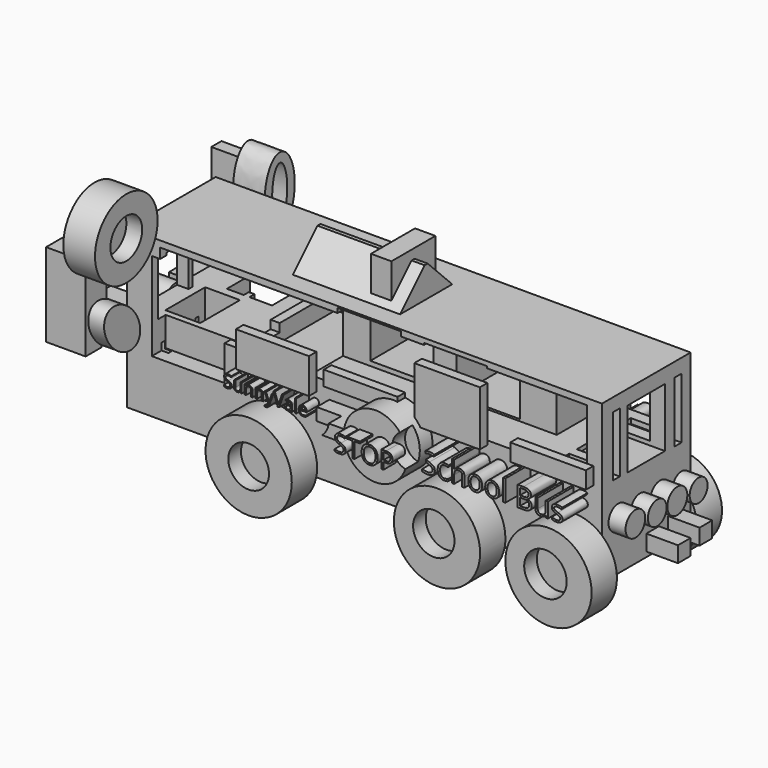
from build123d import *

# Parameters (mm, degrees)
F0_W          = 381
F0_H          = 126.5198698357
F1_DEPTH      = 88.9
F2_W          = 50.8
F2_H          = 50.8
F3_DEPTH      = 127
F4_W          = 50.8
F4_H          = 50.8
F5_DEPTH      = 125.476
F6_W          = 50.8
F6_H          = 50.8
F7_DEPTH      = 353.06
F8_W          = 50.8
F8_H          = 50.8
F9_DEPTH      = 348.996
F10_W         = 36.2219065428
F10_H         = 82.3675262787
F11_DEPTH     = 23.368
F12_W         = 77.2041911259
F12_H         = 49.2639932781
F13_DEPTH     = 88.9
F14_R         = 31.7675639144
F15_DEPTH     = 25.4
F16_R         = 34.5900274771
F17_DEPTH     = 25.4
F18_R         = 34.5948
F19_DEPTH     = 25.4
F20_R         = 34.5948
F21_DEPTH     = 25.4
F22_R         = 34.5948
F23_DEPTH     = 25.4
F24_R         = 34.5948
F25_DEPTH     = 25.4
F26_W         = 58.3547353745
F26_H         = 70.7532842644
F27_DEPTH     = 13.97
F28_W         = 86.0774414614
F28_H         = 53.8219604641
F29_DEPTH     = 24.638
F30_W         = 16.3701735437
F30_H         = 44.1550221294
F31_DEPTH     = 7.62
F32_W         = 12.7
F32_H         = 12.7
F33_DEPTH     = 25.4
F34_W         = 12.7
F34_H         = 12.7
F35_DEPTH     = 25.4
F36_W         = 61.9277469814
F36_H         = 34.5999319106
F37_DEPTH     = 25.4
F38_W         = 4.6026781201
F38_H         = 70.9157045931
F39_DEPTH     = 5.08
F40_W         = 4.1819550097
F40_H         = 60.264851898
F41_DEPTH     = 9.144
F42_W         = 32.3324687779
F42_H         = 9.9669089541
F43_DEPTH     = 25.4
F44_R         = 25.4464837563
F45_DEPTH     = 25.4
F46_W         = 50.8
F46_H         = 5.08
F47_DEPTH     = 25.4
F48_W         = 10.16
F48_H         = 76.2
F49_DEPTH     = 25.4
F51_DEPTH     = 25.4
F52_W         = 142.2856748104
F52_H         = 27.6914052665
F53_DEPTH     = 19.05
F54_R         = 18.3963073453
F55_T4_DEPTH  = 267.5098197727
F56_R         = 9.8577445276
F56_R_2       = 9.3926475971
F56_R_3       = 10.0311781721
F56_R_4       = 8.995280697
F57_DEPTH     = 13.716
F58_T4_DEPTH  = 216.7189372501
F58_T11_DEPTH = 216.7189372501
F58_T17_DEPTH = 216.7189372501
F58_T25_DEPTH = 216.7189372501
F58_T32_DEPTH = 216.7189372501
F59_T4_DEPTH  = 216.7189372501
F59_T10_DEPTH = 216.7189372501
F59_T17_DEPTH = 216.7189372501
F59_T25_DEPTH = 216.7189372501
F59_T31_DEPTH = 216.7189372501
F60_W         = 7.0483535528
F60_H         = 48.1858924031
F60_W_2       = 37.5115424395
F60_H_2       = 47.3481267691
F60_W_3       = 7.0474697277
F60_H_3       = 48.6524347216
F61_DEPTH     = 40.64
F62_W         = 2.7957055718
F62_H         = 33.0349653959
F62_W_2       = 2.7912929654
F62_H_2       = 33.7924696505
F62_W_3       = 2.7886535972
F62_H_3       = 35.0428596139
F62_W_4       = 3.2654814422
F62_H_4       = 35.3162623942
F62_W_5       = 3.2645985484
F62_H_5       = 37.0068624616
F62_W_6       = 3.2628290355
F62_H_6       = 37.7731472254
F62_W_7       = 3.7387758493
F62_H_7       = 37.1046811342
F62_W_8       = 3.2584369183
F62_H_8       = 39.2618253827
F63_DEPTH     = 25.4
F64_R         = 10.9485201538
F65_DEPTH     = 25.4
F66_TEXT_SIZE = 19.9620301525
F67_DEPTH     = 25.4
F68_TEXT_SIZE = 13.9440008853
F69_DEPTH     = 12.7
F70_TEXT_SIZE = 22.4992270685
F71_DEPTH     = 25.4
F72_TEXT_SIZE = 19.452727348
F73_DEPTH     = 12.7
F74_W         = 64.9670958519
F74_H         = 13.338890858
F75_DEPTH     = 31.75
F76_W         = 31.75
F76_H         = 20.7315831661
F77_DEPTH     = 53.594
F78_R         = 31.3869658327
F79_DEPTH     = 25.4
F80_R         = 16.3249163215
F80_R_2       = 16.6206391451
F80_R_3       = 17.0464544412
F80_R_4       = 14.0490359697
F80_R_5       = 15.6096867974
F80_R_6       = 13.548085848
F81_DEPTH     = 12.7
F82_R         = 15.1490274208
F82_R_2       = 15.5967239553
F82_R_3       = 14.1064228958
F83_DEPTH     = 12.7
F84_W         = 68.6886934564
F84_H         = 34.0798477687
F85_DEPTH     = 20.32
F86_R         = 8.4618533599
F87_DEPTH     = 12.7
F88_W         = 58.5370287299
F88_H         = 28.1933201477
F88_W_2       = 59.2209338211
F88_H_2       = 11.8853002787
F88_W_3       = 52.6049807668
F88_H_3       = 43.9174287021
F88_W_4       = 60.577660799
F88_H_4       = 13.7192141265
F89_DEPTH     = 7.62
F90_R         = 12.6748476443
F91_DEPTH     = 7.62
F92_W         = 32.9182857215
F92_H         = 50.8
F93_DEPTH     = 291.846
F94_W         = 55.9817142785
F94_H         = 15.9087059989
F95_DEPTH     = 230.378
F96_W         = 27.9357880354
F96_H         = 39.8813150823
F97_DEPTH     = 25.4
F98_W         = 4.846972879
F98_H         = 34.0798477687
F99_DEPTH     = 25.4
F100_R        = 5.4790358638
F101_DEPTH    = 25.4
F102_R        = 15.9473548046
F103_DEPTH    = 12.7
F105_DEPTH    = 12.7
F106_W        = 7.8915469348
F106_H        = 8.9074093848
F106_W_2      = 8.1563740969
F106_H_2      = 9.9165849388
F107_DEPTH    = 12.7
F109_DEPTH    = 12.7


# Not quite as in the source:
# - a fillet or chamfer that OpenCascade refuses, or shapes differently, is made with other operations: its cross-section is extruded or revolved along the edge and cut away or added
# - Text() gives the source's letters only with a copy of the font that has no kerning and outlines rounded to 1/6400 em; it was checked with that copy


with BuildPart() as f1:
    # F0 (on Front) → F1 (new body)
    with BuildSketch(Plane.XZ):
        with Locations((-29.1106849909, 15.0728300214)):
            Rectangle(F0_W, F0_H)
    extrude(amount=F1_DEPTH)

    # F2 (on face) → F3 (cut)
    with BuildSketch(Plane(origin=(0, 0, 0), x_dir=(-1, 0, 0), z_dir=(0, 1, 0))):
        with Locations((-124.1777315736, 47.8980025902)):
            Rectangle(F2_W, F2_H)
    extrude(amount=-F3_DEPTH, mode=Mode.SUBTRACT)

    # F4 (on face) → F5 (cut)
    with BuildSketch(Plane.XZ.offset(88.9)):
        with Locations((43.9449427649, 49.4133692031)):
            Rectangle(F4_W, F4_H)
    extrude(amount=-F5_DEPTH, mode=Mode.SUBTRACT)

    # F6 (on face) → F7 (cut)
    with BuildSketch(Plane(origin=(0, 0, 0), x_dir=(-1, 0, 0), z_dir=(0, 1, 0))):
        with Locations((25.4, 51.5604968276)):
            Rectangle(F6_W, F6_H)
    extrude(amount=-F7_DEPTH, mode=Mode.SUBTRACT)

    # F8 (on face) → F9 (cut)
    with BuildSketch(Plane(origin=(0, 0, 0), x_dir=(-1, 0, 0), z_dir=(0, 1, 0))):
        with Locations((98.0433411896, 40.8556130676)):
            Rectangle(F8_W, F8_H)
    extrude(amount=-F9_DEPTH, mode=Mode.SUBTRACT)

    # F10 (on face) → F11 (cut)
    with BuildSketch(Plane(origin=(0, 0, 0), x_dir=(-1, 0, 0), z_dir=(0, 1, 0))):
        with Locations((173.8056764007, -7.0033417571)):
            Rectangle(F10_W, F10_H)
    extrude(amount=-F11_DEPTH, mode=Mode.SUBTRACT)

    # F12 (on face) → F13 (cut)
    with BuildSketch(Plane(origin=(-219.6106849909, 0, 0), x_dir=(0, -1, 0), z_dir=(-1, 0, 0))):
        with Locations((43.8935565762, 42.518469505)):
            Rectangle(F12_W, F12_H)
    extrude(amount=-F13_DEPTH, mode=Mode.SUBTRACT)

    # F14 (on face) → F15 (join)
    with BuildSketch(Plane(origin=(0, 0, 0), x_dir=(-1, 0, 0), z_dir=(0, 1, 0))):
        with Locations((-134.4692409039, -42.1050563455)):
            Circle(F14_R)
    extrude(amount=F15_DEPTH)

    # F16 (on face) → F17 (join)
    with BuildSketch(Plane(origin=(0, 0, 0), x_dir=(-1, 0, 0), z_dir=(0, 1, 0))):
        with Locations((-54.2609095573, -41.1995537579)):
            Circle(F16_R)
    extrude(amount=F17_DEPTH)

    # F18 (on face) → F19 (join)
    with BuildSketch(Plane(origin=(0, 0, 0), x_dir=(-1, 0, 0), z_dir=(0, 1, 0))):
        with Locations((101.8479317427, -41.1263331771)):
            Circle(F18_R)
    extrude(amount=F19_DEPTH)

    # F20 (on face) → F21 (join)
    with BuildSketch(Plane.XZ.offset(88.9)):
        with Locations((138.8085335493, -40.9661456943)):
            Circle(F20_R)
    extrude(amount=F21_DEPTH)

    # F22 (on face) → F23 (join)
    with BuildSketch(Plane.XZ.offset(88.9)):
        with Locations((49.349758774, -42.1094596386)):
            Circle(F22_R)
    extrude(amount=F23_DEPTH)

    # F24 (on face) → F25 (join)
    with BuildSketch(Plane.XZ.offset(88.9)):
        with Locations((-101.7133966088, -41.3157492876)):
            Circle(F24_R)
    extrude(amount=F25_DEPTH)

    # F26 (on face) → F27 (cut)
    with BuildSketch(Plane.XZ.offset(88.9)):
        with Locations((-170.5612689257, 29.7877525445)):
            Rectangle(F26_W, F26_H)
    extrude(amount=-F27_DEPTH, mode=Mode.SUBTRACT)

    # F28 (on face) → F29 (join)
    with BuildSketch(Plane.XY.offset(78.3327649392)):
        with Locations((-56.0307926498, -47.2026942298)):
            Rectangle(F28_W, F28_H)
    extrude(amount=F29_DEPTH)

    # F30 (on face) → F31 (join)
    with BuildSketch(Plane.XY.offset(102.9707649392)):
        with Locations((-31.680950895, -46.8696849421)):
            Rectangle(F30_W, F30_H)
    extrude(amount=F31_DEPTH)

    # F32 (on face) → F33 (join)
    with BuildSketch(Plane.YZ.offset(161.3893150091)):
        with Locations((-16.4386960678, -34.2422378585)):
            Rectangle(F32_W, F32_H)
    extrude(amount=F33_DEPTH)

    # F34 (on face) → F35 (join)
    with BuildSketch(Plane.YZ.offset(161.3893150091)):
        with Locations((-38.1, -37.8550173879)):
            Rectangle(F34_W, F34_H)
    extrude(amount=F35_DEPTH)

    # F36 (on face) → F37 (cut)
    with BuildSketch(Plane(origin=(-130.7106849909, 0, 0), x_dir=(0, -1, 0), z_dir=(-1, 0, 0))):
        with Locations((40.43697007, 46.5236147866)):
            Rectangle(F36_W, F36_H)
    extrude(amount=-F37_DEPTH, mode=Mode.SUBTRACT)

    # F38 (on face) → F39 (join)
    with BuildSketch(Plane(origin=(0, -23.368, 0), x_dir=(-1, 0, 0), z_dir=(0, 1, 0))):
        with Locations((176.1070154607, -17.5713794306)):
            Rectangle(F38_W, F38_H)
    extrude(amount=F39_DEPTH)

    # F40 (on face) → F41 (join)
    with BuildSketch(Plane(origin=(-219.6106849909, 0, 0), x_dir=(0, -1, 0), z_dir=(-1, 0, 0))):
        with Locations((36.5860965103, 42.0981813222)):
            Rectangle(F40_W, F40_H)
    extrude(amount=-F41_DEPTH)

    # F42 (on face) → F43 (join)
    with BuildSketch(Plane.XZ.offset(88.9)):
        with Locations((-41.1809217185, 4.983454477)):
            Rectangle(F42_W, F42_H)
    extrude(amount=F43_DEPTH)

    # F44 (on face) → F45 (join)
    with BuildSketch(Plane.XZ.offset(88.9)):
        with Locations((0, 6.0606561601)):
            Circle(F44_R)
    extrude(amount=F45_DEPTH)

    # F46 (on face) → F47 (join)
    with BuildSketch(Plane(origin=(-219.6106849909, 0, 0), x_dir=(0, -1, 0), z_dir=(-1, 0, 0))):
        with Locations((-10.1813804358, 6.5084572987)):
            Rectangle(F46_W, F46_H)
    extrude(amount=F47_DEPTH)

    # F48 (on face) → F49 (join)
    with BuildSketch(Plane(origin=(-245.0106849909, 0, 0), x_dir=(0, -1, 0), z_dir=(-1, 0, 0))):
        with Locations((-32.4664697665, 42.0684572987)):
            Rectangle(F48_W, F48_H)
    extrude(amount=-F49_DEPTH)

    # F50 (on face) → F51 (join)
    with BuildSketch(Plane.YZ.offset(-219.6106849909)):
        with BuildLine():
            add(Edge.make_bspline(
                [(32.4664697665, 90.7859504223), (6.4393695077, 90.7859504223), (19.4529196371, 49.0357801318), (32.4664697665, 7.2856098413), (45.4800198959, 49.0357801318), (58.4935700253, 90.7859504223), (32.4664697665, 90.7859504223)],
                knots=[0, 0, 0, 2.0943951024, 2.0943951024, 4.1887902048, 4.1887902048, 6.2831853072, 6.2831853072, 6.2831853072], degree=2, weights=[1, 0.5, 1, 0.5, 1, 0.5, 1]))
        make_face()
    extrude(amount=F51_DEPTH)

    # F52 (on face) → F53 (join)
    with BuildSketch(Plane(origin=(0, 0, -48.1871048965), x_dir=(1, 0, 0), z_dir=(0, 0, -1))):
        with Locations((71.1428374052, 47.2517032176)):
            Rectangle(F52_W, F52_H)
    extrude(amount=F53_DEPTH)

    # F54
    f54_edges = [f1.edges().sort_by_distance(p)[0] for p in [
        (142.285675, -47.251703, -67.237105),
    ]]
    fillet(f54_edges, radius=F54_R)

    # F55: fillet of radius 69.9059679121 on 1 edges, made by hand


with BuildPart() as f55_tool2:
    # F55_s3 → F55_t4 (new body)
    with BuildSketch(Plane.XZ.offset(181.006613104)):
        with BuildLine():
            ThreePointArc((47.9636829012, -67.2371048965), (22.1595292751, -62.3002835492), (0, -48.1871048965))
            Line((0, -48.1871048965), (0, -67.2371048965))
            Line((0, -67.2371048965), (47.9636829012, -67.2371048965))
        make_face()
    extrude(amount=-F55_T4_DEPTH)

    split(bisect_by=Plane.XZ.offset(88.9), keep=Keep.BOTTOM)

    split(bisect_by=Plane.XZ, keep=Keep.TOP)


with BuildPart() as f1_1:
    add(f1.part)

    # F55_t1: cut F55_tool2
    add(f55_tool2.part, mode=Mode.SUBTRACT)

    # F56 (on face) → F57 (join)
    with BuildSketch(Plane.YZ.offset(161.3893150091)):
        with Locations((-72.517581284, -8.7204622105)):
            Circle(F56_R)
        with Locations((-50.6030321121, -9.8998090252)):
            Circle(F56_R_2)
        with Locations((-30.4931569844, -9.6532292664)):
            Circle(F56_R_3)
        with Locations((-9.1150775552, -10.8976587653)):
            Circle(F56_R_4)
    extrude(amount=F57_DEPTH)

    # F58: chamfer of 25.4 on 1 edges, made by hand


with BuildPart() as f58_tool2:
    # F58_s3 → F58_t4 (new body)
    with BuildSketch(Plane.YZ.offset(-164.3902612749)):
        Polygon((-74.1136744618, 77.5707649392), (-48.7136744618, 102.9707649392), (-74.1136744618, 102.9707649392), align=None)
    extrude(amount=F58_T4_DEPTH)

    split(bisect_by=Plane.XY.offset(78.3327649392), keep=Keep.TOP)

    split(bisect_by=Plane.YZ.offset(-39.8660376668), keep=Keep.BOTTOM)

    split(bisect_by=Plane.XZ.offset(68.9471960068), keep=Keep.TOP)


with BuildPart() as f1_2:
    add(f1_1.part)

    # F58_t1: cut F58_tool2
    add(f58_tool2.part, mode=Mode.SUBTRACT)


with BuildPart() as f58_tool9:
    # F58_s10 → F58_t11 (new body)
    with BuildSketch(Plane.YZ.offset(-164.3902612749)):
        Polygon((-74.1136744618, 77.5707649392), (-48.7136744618, 102.9707649392), (-74.1136744618, 102.9707649392), align=None)
    extrude(amount=F58_T11_DEPTH)

    split(bisect_by=Plane.YZ.offset(-39.8660376668), keep=Keep.BOTTOM)

    split(bisect_by=Plane.XZ.offset(68.9471960068), keep=Keep.BOTTOM)


with BuildPart() as f1_3:
    add(f1_2.part)

    # F58_t8: cut F58_tool9
    add(f58_tool9.part, mode=Mode.SUBTRACT)


with BuildPart() as f58_tool15:
    # F58_s16 → F58_t17 (new body)
    with BuildSketch(Plane.YZ.offset(-164.3902612749)):
        Polygon((-74.1136744618, 77.5707649392), (-48.7136744618, 102.9707649392), (-74.1136744618, 102.9707649392), align=None)
    extrude(amount=F58_T17_DEPTH)

    split(bisect_by=Plane.XY.offset(78.3327649392), keep=Keep.TOP)

    split(bisect_by=Plane.YZ.offset(-39.8660376668), keep=Keep.TOP)

    split(bisect_by=Plane.XZ.offset(68.9471960068), keep=Keep.TOP)

    split(bisect_by=Plane.YZ.offset(-23.4958641231), keep=Keep.BOTTOM)


with BuildPart() as f1_4:
    add(f1_3.part)

    # F58_t14: cut F58_tool15
    add(f58_tool15.part, mode=Mode.SUBTRACT)


with BuildPart() as f58_tool23:
    # F58_s24 → F58_t25 (new body)
    with BuildSketch(Plane.YZ.offset(-164.3902612749)):
        Polygon((-74.1136744618, 77.5707649392), (-48.7136744618, 102.9707649392), (-74.1136744618, 102.9707649392), align=None)
    extrude(amount=F58_T25_DEPTH)

    split(bisect_by=Plane.XY.offset(78.3327649392), keep=Keep.TOP)

    split(bisect_by=Plane.XZ.offset(68.9471960068), keep=Keep.TOP)

    split(bisect_by=Plane.YZ.offset(-23.4958641231), keep=Keep.TOP)


with BuildPart() as f1_5:
    add(f1_4.part)

    # F58_t22: cut F58_tool23
    add(f58_tool23.part, mode=Mode.SUBTRACT)


with BuildPart() as f58_tool30:
    # F58_s31 → F58_t32 (new body)
    with BuildSketch(Plane.YZ.offset(-164.3902612749)):
        Polygon((-74.1136744618, 77.5707649392), (-48.7136744618, 102.9707649392), (-74.1136744618, 102.9707649392), align=None)
    extrude(amount=F58_T32_DEPTH)

    split(bisect_by=Plane.XZ.offset(68.9471960068), keep=Keep.BOTTOM)

    split(bisect_by=Plane.YZ.offset(-23.4958641231), keep=Keep.TOP)


with BuildPart() as f1_6:
    add(f1_5.part)

    # F58_t29: cut F58_tool30
    add(f58_tool30.part, mode=Mode.SUBTRACT)

    # F59: chamfer of 25.4 on 1 edges, made by hand


with BuildPart() as f59_tool2:
    # F59_s3 → F59_t4 (new body)
    with BuildSketch(Plane.YZ.offset(52.3286759752)):
        Polygon((-45.6917139977, 102.9707649392), (-20.2917139977, 77.5707649392), (-20.2917139977, 102.9707649392), align=None)
    extrude(amount=-F59_T4_DEPTH)

    split(bisect_by=Plane.YZ.offset(-23.4958641231), keep=Keep.TOP)

    split(bisect_by=Plane.XZ.offset(24.7921738774), keep=Keep.TOP)


with BuildPart() as f1_7:
    add(f1_6.part)

    # F59_t1: cut F59_tool2
    add(f59_tool2.part, mode=Mode.SUBTRACT)


with BuildPart() as f59_tool8:
    # F59_s9 → F59_t10 (new body)
    with BuildSketch(Plane.YZ.offset(52.3286759752)):
        Polygon((-45.6917139977, 102.9707649392), (-20.2917139977, 77.5707649392), (-20.2917139977, 102.9707649392), align=None)
    extrude(amount=-F59_T10_DEPTH)

    split(bisect_by=Plane.XY.offset(78.3327649392), keep=Keep.TOP)

    split(bisect_by=Plane.YZ.offset(-23.4958641231), keep=Keep.TOP)

    split(bisect_by=Plane.XZ.offset(24.7921738774), keep=Keep.BOTTOM)


with BuildPart() as f1_8:
    add(f1_7.part)

    # F59_t7: cut F59_tool8
    add(f59_tool8.part, mode=Mode.SUBTRACT)


with BuildPart() as f59_tool15:
    # F59_s16 → F59_t17 (new body)
    with BuildSketch(Plane.YZ.offset(52.3286759752)):
        Polygon((-45.6917139977, 102.9707649392), (-20.2917139977, 77.5707649392), (-20.2917139977, 102.9707649392), align=None)
    extrude(amount=-F59_T17_DEPTH)

    split(bisect_by=Plane.XY.offset(78.3327649392), keep=Keep.TOP)

    split(bisect_by=Plane.YZ.offset(-23.4958641231), keep=Keep.BOTTOM)

    split(bisect_by=Plane.XZ.offset(24.7921738774), keep=Keep.BOTTOM)

    split(bisect_by=Plane.YZ.offset(-39.8660376668), keep=Keep.TOP)


with BuildPart() as f1_9:
    add(f1_8.part)

    # F59_t14: cut F59_tool15
    add(f59_tool15.part, mode=Mode.SUBTRACT)


with BuildPart() as f59_tool23:
    # F59_s24 → F59_t25 (new body)
    with BuildSketch(Plane.YZ.offset(52.3286759752)):
        Polygon((-45.6917139977, 102.9707649392), (-20.2917139977, 77.5707649392), (-20.2917139977, 102.9707649392), align=None)
    extrude(amount=-F59_T25_DEPTH)

    split(bisect_by=Plane.XZ.offset(24.7921738774), keep=Keep.TOP)

    split(bisect_by=Plane.YZ.offset(-39.8660376668), keep=Keep.BOTTOM)


with BuildPart() as f1_10:
    add(f1_9.part)

    # F59_t22: cut F59_tool23
    add(f59_tool23.part, mode=Mode.SUBTRACT)


with BuildPart() as f59_tool29:
    # F59_s30 → F59_t31 (new body)
    with BuildSketch(Plane.YZ.offset(52.3286759752)):
        Polygon((-45.6917139977, 102.9707649392), (-20.2917139977, 77.5707649392), (-20.2917139977, 102.9707649392), align=None)
    extrude(amount=-F59_T31_DEPTH)

    split(bisect_by=Plane.XY.offset(78.3327649392), keep=Keep.TOP)

    split(bisect_by=Plane.XZ.offset(24.7921738774), keep=Keep.BOTTOM)

    split(bisect_by=Plane.YZ.offset(-39.8660376668), keep=Keep.BOTTOM)


with BuildPart() as f1_11:
    add(f1_10.part)

    # F59_t28: cut F59_tool29
    add(f59_tool29.part, mode=Mode.SUBTRACT)

    # F60 (on face) → F61 (cut)
    with BuildSketch(Plane.YZ.offset(161.3893150091)):
        with Locations((-74.5554566383, 43.6637960374)):
            Rectangle(F60_W, F60_H)
        with Locations((-44.5713028312, 42.8774356842)):
            Rectangle(F60_W_2, F60_H_2)
        with Locations((-12.682036031, 42.755770497)):
            Rectangle(F60_W_3, F60_H_3)
    extrude(amount=-F61_DEPTH, mode=Mode.SUBTRACT)

    # F62 (on face) → F63 (cut)
    with BuildSketch(Plane(origin=(-219.6106849909, 0, 0), x_dir=(0, -1, 0), z_dir=(-1, 0, 0))):
        with Locations((10.113844648, -16.517482698)):
            Rectangle(F62_W, F62_H)
        with Locations((19.6323245764, -16.8962348253)):
            Rectangle(F62_W_2, F62_H_2)
        with Locations((27.7247251943, -17.5214298069)):
            Rectangle(F62_W_3, F62_H_3)
        with Locations((38.4348314255, -17.6581311971)):
            Rectangle(F62_W_4, F62_H_4)
        with Locations((47.9568392038, -18.5034312308)):
            Rectangle(F62_W_5, F62_H_5)
        with Locations((57.0006947964, -18.8865736127)):
            Rectangle(F62_W_6, F62_H_6)
        with Locations((68.1845396757, -18.5523405671)):
            Rectangle(F62_W_7, F62_H_7)
        with Locations((77.4676948786, -19.6309126914)):
            Rectangle(F62_W_8, F62_H_8)
    extrude(amount=-F63_DEPTH, mode=Mode.SUBTRACT)

    # F64 (on face) → F65 (join)
    with BuildSketch(Plane(origin=(-219.6106849909, 0, 0), x_dir=(0, -1, 0), z_dir=(-1, 0, 0))):
        with Locations((40.0675721467, 8.8824788108)):
            Circle(F64_R)
    extrude(amount=F65_DEPTH)

    # F66 (on face) → F67 (join)
    with BuildSketch(Plane(origin=(0, 0, 0), x_dir=(-1, 0, 0), z_dir=(0, 1, 0))):
        with Locations((-112.6251146197, 0)):
            Text('SunnyVale School Bus', F66_TEXT_SIZE, font='Open Sans', text_align=(TextAlign.LEFT, TextAlign.BOTTOM))
    extrude(amount=F67_DEPTH)

    # F68 (on face) → F69 (join)
    with BuildSketch(Plane.XZ.offset(88.9)):
        with Locations((-132.4551999569, 0)):
            Text('SunnyVale', F68_TEXT_SIZE, font='Open Sans', text_align=(TextAlign.LEFT, TextAlign.BOTTOM))
    extrude(amount=F69_DEPTH)

    # F70 (on face) → F71 (join)
    with BuildSketch(Plane.XZ.offset(88.9)):
        with Locations((36.3434664905, 0)):
            Text('School Bus', F70_TEXT_SIZE, font='Open Sans', text_align=(TextAlign.LEFT, TextAlign.BOTTOM))
    extrude(amount=F71_DEPTH)

    # F72 (on face) → F73 (join)
    with BuildSketch(Plane.XZ.offset(114.3)):
        with Locations((-23.5150475055, 0)):
            Text('STOP', F72_TEXT_SIZE, font='Open Sans', text_align=(TextAlign.LEFT, TextAlign.BOTTOM))
    extrude(amount=F73_DEPTH)

    # F74 (on face) → F75 (join)
    with BuildSketch(Plane(origin=(-219.6106849909, 0, 0), x_dir=(0, -1, 0), z_dir=(-1, 0, 0))):
        with Locations((97.8796184063, 11.2170274369)):
            Rectangle(F74_W, F74_H)
    extrude(amount=F75_DEPTH)

    # F76 (on face) → F77 (join)
    with BuildSketch(Plane.XY.offset(17.8864728659)):
        with Locations((-235.4856849909, -119.9973747492)):
            Rectangle(F76_W, F76_H)
    extrude(amount=F77_DEPTH)

    # F78 (on face) → F79 (join)
    with BuildSketch(Plane.YZ.offset(-219.6106849909)):
        with Locations((-121.3685572147, 92.4738794565)):
            Circle(F78_R)
    extrude(amount=F79_DEPTH)

    # F80 (on face) → F81 (cut)
    with BuildSketch(Plane.XZ.offset(114.3)):
        with Locations((-101.7133966088, -41.3157492876)):
            Circle(F80_R)
        with Locations((46.8045808375, -40.3528511524)):
            Circle(F80_R_2)
        with Locations((136.3797336817, -39.8180782795)):
            Circle(F80_R_3)
        with Locations((-211.3364040852, 8.7373647839)):
            Circle(F80_R_4)
        with Locations((-52.9816895723, 11.771232821)):
            Circle(F80_R_5)
        with Locations((27.1298289299, 10.9193101525)):
            Circle(F80_R_6)
    extrude(amount=-F81_DEPTH, mode=Mode.SUBTRACT)

    # F82 (on face) → F83 (cut)
    with BuildSketch(Plane(origin=(0, 25.4, 0), x_dir=(-1, 0, 0), z_dir=(0, 1, 0))):
        with Locations((-134.4692409039, -42.1050563455)):
            Circle(F82_R)
        with Locations((-58.2725554705, -40.8917069435)):
            Circle(F82_R_2)
        with Locations((100.4514545202, -38.7619435787)):
            Circle(F82_R_3)
    extrude(amount=-F83_DEPTH, mode=Mode.SUBTRACT)

    # F84 (on face) → F85 (join)
    with BuildSketch(Plane(origin=(0, 0, 0), x_dir=(-1, 0, 0), z_dir=(0, 1, 0))):
        with Locations((23.6279056408, -31.1471810121)):
            Rectangle(F84_W, F84_H)
    extrude(amount=F85_DEPTH)

    # F86 (on face) → F87 (join)
    with BuildSketch(Plane(origin=(0, 20.32, 0), x_dir=(-1, 0, 0), z_dir=(0, 1, 0))):
        with Locations((40.0207266212, -25.0336714089)):
            Circle(F86_R)
    extrude(amount=F87_DEPTH)

    # F88 (on face) → F89 (join)
    with BuildSketch(Plane.XZ.offset(88.9)):
        with Locations((-96.896160394, 26.374051813)):
            Rectangle(F88_W, F88_H)
        with Locations((-26.1106782127, 28.9179570973)):
            Rectangle(F88_W_2, F88_H_2)
        with Locations((43.2074554265, 41.1041397601)):
            Rectangle(F88_W_3, F88_H_3)
        with Locations((124.2348402739, 25.2086902037)):
            Rectangle(F88_W_4, F88_H_4)
    extrude(amount=F89_DEPTH)

    # F90 (on face) → F91 (join)
    with BuildSketch(Plane(origin=(0, 0, 0), x_dir=(-1, 0, 0), z_dir=(0, 1, 0))):
        with Locations((-137.7950459719, 4.4631408527)):
            Circle(F90_R)
    extrude(amount=F91_DEPTH)

    # F92 (on face) → F93 (cut)
    with BuildSketch(Plane.YZ.offset(98.7777315736)):
        with Locations((-72.4408571392, 47.8980025902)):
            Rectangle(F92_W, F92_H)
    extrude(amount=-F93_DEPTH, mode=Mode.SUBTRACT)

    # F94 (on face) → F95 (cut)
    with BuildSketch(Plane.YZ.offset(98.7777315736)):
        with Locations((-27.9908571392, 65.3436495907)):
            Rectangle(F94_W, F94_H)
    extrude(amount=-F95_DEPTH, mode=Mode.SUBTRACT)

    # F96 (on face) → F97 (cut)
    with BuildSketch(Plane.XY.offset(17.8864728659)):
        with Locations((-189.9014934897, -50.1457992941)):
            Rectangle(F96_W, F96_H)
    extrude(amount=-F97_DEPTH, mode=Mode.SUBTRACT)

    # F98 (on face) → F99 (cut)
    with BuildSketch(Plane(origin=(0, 20.32, 0), x_dir=(-1, 0, 0), z_dir=(0, 1, 0))):
        with Locations((26.0513920803, -31.1471810121)):
            Rectangle(F98_W, F98_H)
    extrude(amount=-F99_DEPTH, mode=Mode.SUBTRACT)

    # F100 (on face) → F101 (join)
    with BuildSketch(Plane(origin=(0, 20.32, 0), x_dir=(-1, 0, 0), z_dir=(0, 1, 0))):
        with Locations((15.9555636346, -24.342238903)):
            Circle(F100_R)
    extrude(amount=F101_DEPTH)

    # F102 (on face) → F103 (cut)
    with BuildSketch(Plane.YZ.offset(-194.2106849909)):
        with Locations((-121.3685572147, 92.4738794565)):
            Circle(F102_R)
    extrude(amount=-F103_DEPTH, mode=Mode.SUBTRACT)

    # F104 (on face) → F105 (cut)
    with BuildSketch(Plane.YZ.offset(-194.2106849909)):
        with BuildLine():
            add(Edge.make_bspline(
                [(32.4664697665, 83.3176672459), (19.4137892698, 83.3176672459), (25.9401295181, 52.76992172), (32.4664697665, 22.2221761942), (38.9928100148, 52.76992172), (45.5191502632, 83.3176672459), (32.4664697665, 83.3176672459)],
                knots=[0, 0, 0, 2.0943951024, 2.0943951024, 4.1887902048, 4.1887902048, 6.2831853072, 6.2831853072, 6.2831853072], degree=2, weights=[1, 0.5, 1, 0.5, 1, 0.5, 1]))
        make_face()
    extrude(amount=-F105_DEPTH, mode=Mode.SUBTRACT)

    # F106 (on face) → F107 (join)
    with BuildSketch(Plane(origin=(0, 0, -48.1871048965), x_dir=(1, 0, 0), z_dir=(0, 0, -1))):
        with Locations((-54.0264789015, 19.871561788)):
            Rectangle(F106_W, F106_H)
        with Locations((-48.462420702, 51.6203362495)):
            Rectangle(F106_W_2, F106_H_2)
    extrude(amount=F107_DEPTH)

    # F108 (on face) → F109 (join)
    with BuildSketch(Plane.YZ.offset(-219.6106849909)):
        with BuildLine():
            add(Edge.make_bspline(
                [(-124.7065365314, 36.4932306111), (-142.1310318848, 20.4784485794), (-110.8063541602, 3.8829332603), (-79.4816764355, -12.7125820589), (-93.3818588068, 19.8977152919), (-107.2820411781, 52.5080126427), (-124.7065365314, 36.4932306111)],
                knots=[0, 0, 0, 2.0943951024, 2.0943951024, 4.1887902048, 4.1887902048, 6.2831853072, 6.2831853072, 6.2831853072], degree=2, weights=[1, 0.5, 1, 0.5, 1, 0.5, 1]))
        make_face()
    extrude(amount=F109_DEPTH)


solid = f1_11.part
